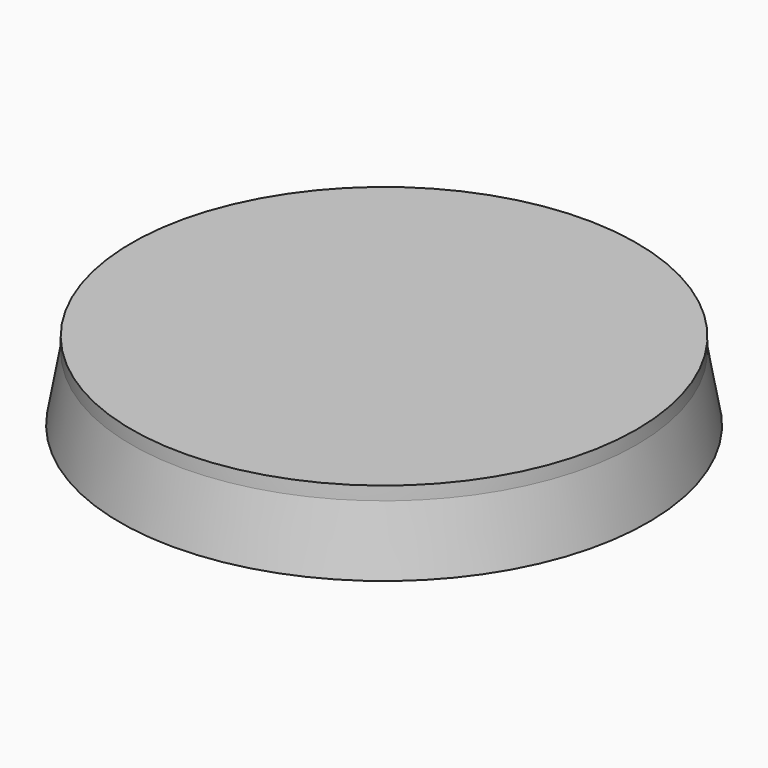
from build123d import *

# Parameters (mm, degrees)
F3_R             = 37.5
F4_DEPTH         = 2
F7_R             = 2.5
F8_DEPTH         = 5
F8_TAPER         = 2
F12_COPIES_COUNT = 2
F14_COPIES_COUNT = 2


# Not quite as in the source:
# - a pattern or mirror of a feature is missing from the dataset's text; its kind, count and spacing are read off the source's solid


with BuildPart() as f2:
    # F1 (on Front) → F2 (revolve)
    with BuildSketch(Plane.XZ):
        with BuildLine():
            Line((-16, 0), (-21.33, 0))
            ThreePointArc((-21.33, 0), (-18.665, -2.665), (-16, 0))
        make_face()
    revolve(axis=Axis((0, 0, 18.396249041), (0, 0, 1)))

    # F3 (on face) → F4 (join)
    with BuildSketch(Plane.XY):
        Circle(F3_R)
    extrude(amount=F4_DEPTH)

    # F5 (on Right) → F6 (revolve)
    with BuildSketch(Plane.YZ):
        Polygon((-36.8366060944, -9.6), (-35.1438670796, 0), (-37.5, 0), (-39.1927390148, -9.6), align=None)
    revolve(axis=Axis((0, 0, 18.396249041), (0, 0, 1)))

    # F7 (on face) → F8 (join)
    with BuildSketch(Plane(origin=(0, 0, 0), x_dir=(1, 0, 0), z_dir=(0, 0, -1))):
        with Locations((0, 30.5)):
            Circle(F7_R)
        with Locations((-26.4137748154, -15.25)):
            Circle(F7_R)
        with Locations((26.4137748154, -15.25)):
            Circle(F7_R)
    extrude(amount=F8_DEPTH, taper=F8_TAPER)

    # F11 (on offset) → F12 (join, up to the next surface of F2)
    with BuildSketch(Plane.YZ.offset(33)):
        with BuildLine():
            Line((2.5, 0), (-2.5, 0))
            ThreePointArc((-2.5, 0), (0, -2.5), (2.5, 0))
        make_face()
    f12 = extrude(until=Until.NEXT)

    # F12_copies: F12 ×2 about axis
    f12_copies_axis = Axis((0, 0, 0), (0, 0, 1))
    for i in range(1, F12_COPIES_COUNT):
        add(f12.rotate(f12_copies_axis, i * 360 / F12_COPIES_COUNT))

    # F13 (on offset) → F14 (join, up to the next surface of F2)
    with BuildSketch(Plane.YZ.offset(23)):
        with BuildLine():
            Line((1, 0), (-1, 0))
            ThreePointArc((-1, 0), (0, -1), (1, 0))
        make_face()
    f14 = extrude(until=Until.NEXT, dir=(-1, 0, 0))

    # F14_copies: F14 ×2 about axis
    f14_copies_axis = Axis((0, 0, 0), (0, 0, 1))
    for i in range(1, F14_COPIES_COUNT):
        add(f14.rotate(f14_copies_axis, i * 360 / F14_COPIES_COUNT))

    # F14_face (on face) → F15 section 0
    with BuildSketch(Plane(origin=(23, 0, -0.4244131816), x_dir=(0, 1, 0), z_dir=(1, 0, 0))):
        with BuildLine():
            Line((1, 0.4244131816), (-1, 0.4244131816))
            ThreePointArc((-1, 0.4244131816), (0, -0.5755868184), (1, 0.4244131816))
        make_face()
    # F12_face (on face) → F15 section 1
    with BuildSketch(Plane(origin=(33, 0, -1.0610329539), x_dir=(0, 1, 0), z_dir=(-1, 0, 0))):
        with BuildLine():
            Line((-2.5, -1.0610329539), (2.5, -1.0610329539))
            ThreePointArc((2.5, -1.0610329539), (0, 1.4389670461), (-2.5, -1.0610329539))
        make_face()
    f15 = loft()

    # F15_copies: F15 across plane
    add(f15.mirror(Plane(origin=(0, 0, 0), x_dir=(0, 0, -1), z_dir=(-1, 0, 0))))


solid = f2.part
